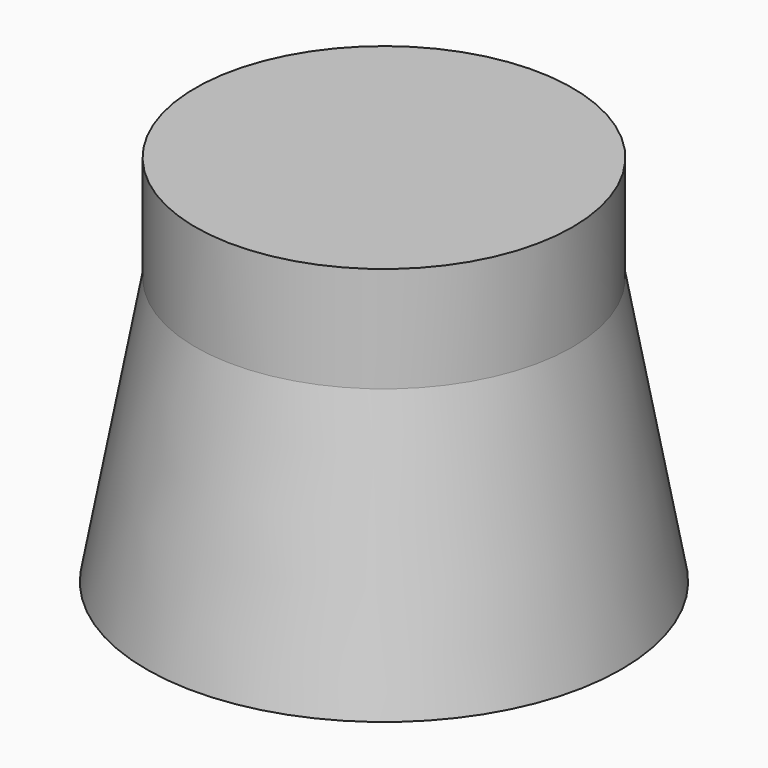
from build123d import *

# Parameters (mm, degrees)
F0_R     = 31.5
F2_R     = 25
F4_DEPTH = 14


with BuildPart() as f3:
    # F0 (on Top) → F3 section 0
    with BuildSketch(Plane.XY):
        Circle(F0_R)
    # F2 (on offset) → F3 section 1
    with BuildSketch(Plane.XY.offset(35.5)):
        Circle(F2_R)
    loft()


with BuildPart() as f4:
    # F4 (new): a face of the model
    f4_faces = [f3.part.faces().sort_by_distance(p)[0] for p in [
        (0, 0, 35.5),
    ]]
    extrude(f4_faces, amount=F4_DEPTH)


solid = Compound([f3.part, f4.part])
